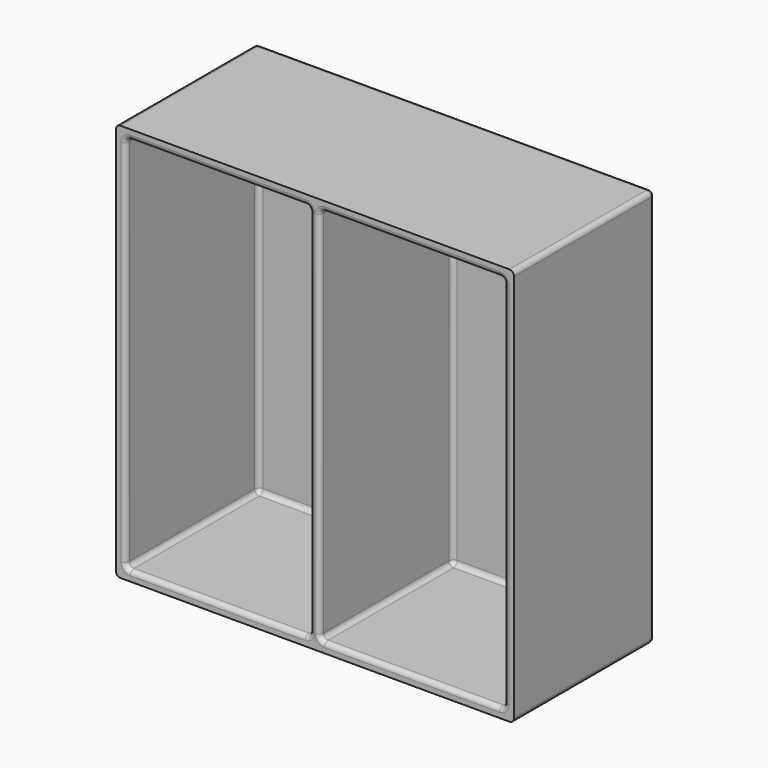
from build123d import *

# Parameters (mm, degrees)
F0_W     = 129.54
F0_H     = 129.54
F1_DEPTH = 57.15
F2_T     = -3.175
F3_R     = 1.524
F4_R     = 1.524
F5_W     = 3.175
F5_H     = 1.524
F5_H_2   = 120.142
F6_DEPTH = 53.975
F7_R     = 1.524


with BuildPart() as f1:
    # F0 (on Front) → F1 (new body)
    with BuildSketch(Plane.XZ):
        with Locations((64.77, 64.77)):
            Rectangle(F0_W, F0_H)
    extrude(amount=-F1_DEPTH)

    # F2
    f2_openings = [f1.faces().sort_by_distance(p)[0] for p in [
        (64.77, 0, 64.77),
    ]]
    offset(amount=F2_T, openings=f2_openings)

    # F3
    f3_edges = [f1.edges().sort_by_distance(p)[0] for p in [
        (3.175, 26.9875, 126.365),
        (64.77, 53.975, 126.365),
        (3.175, 53.975, 64.77),
        (3.175, 26.9875, 3.175),
        (64.77, 53.975, 3.175),
        (126.365, 53.975, 64.77),
        (126.365, 26.9875, 126.365),
        (126.365, 26.9875, 3.175),
    ]]
    fillet(f3_edges, radius=F3_R)

    # F4
    f4_edges = [f1.edges().sort_by_distance(p)[0] for p in [
        (129.54, 28.575, 0),
        (64.77, 57.15, 0),
        (129.54, 57.15, 64.77),
        (129.54, 28.575, 129.54),
        (64.77, 57.15, 129.54),
        (0, 28.575, 129.54),
        (0, 57.15, 64.77),
        (0, 28.575, 0),
    ]]
    fillet(f4_edges, radius=F4_R)

    # F5 (on face) → F6 (join)
    with BuildSketch(Plane.XZ.offset(-53.975)):
        with Locations((64.77, 125.603)):
            Rectangle(F5_W, F5_H)
        with Locations((64.77, 64.77)):
            Rectangle(F5_W, F5_H_2)
        with Locations((64.77, 3.937)):
            Rectangle(F5_W, F5_H)
    extrude(amount=F6_DEPTH)

    # F7
    f7_edges = [f1.edges().sort_by_distance(p)[0] for p in [
        (33.94075, 0, 126.365),
        (63.1825, 0, 64.77),
        (63.1825, 53.528631, 125.918631),
        (63.1825, 53.975, 64.77),
        (63.1825, 53.528631, 3.621369),
        (63.1825, 26.2255, 3.175),
        (63.1825, 26.2255, 126.365),
        (95.59925, 0, 126.365),
        (66.3575, 26.2255, 126.365),
        (95.59925, 52.451, 126.365),
        (124.841, 26.2255, 126.365),
        (126.365, 0, 64.77),
        (126.365, 26.2255, 4.699),
        (126.365, 26.2255, 124.841),
        (126.365, 52.451, 64.77),
        (3.175, 0, 64.77),
        (3.621369, 0, 125.918631),
        (33.94075, 0, 3.175),
        (3.621369, 0, 3.621369),
        (125.918631, 0, 125.918631),
        (125.918631, 0, 3.621369),
        (95.59925, 0, 3.175),
        (66.3575, 0, 64.77),
        (66.3575, 26.2255, 3.175),
        (66.3575, 53.528631, 3.621369),
        (66.3575, 53.975, 64.77),
        (66.3575, 53.528631, 125.918631),
    ]]
    fillet(f7_edges, radius=F7_R)


solid = f1.part
